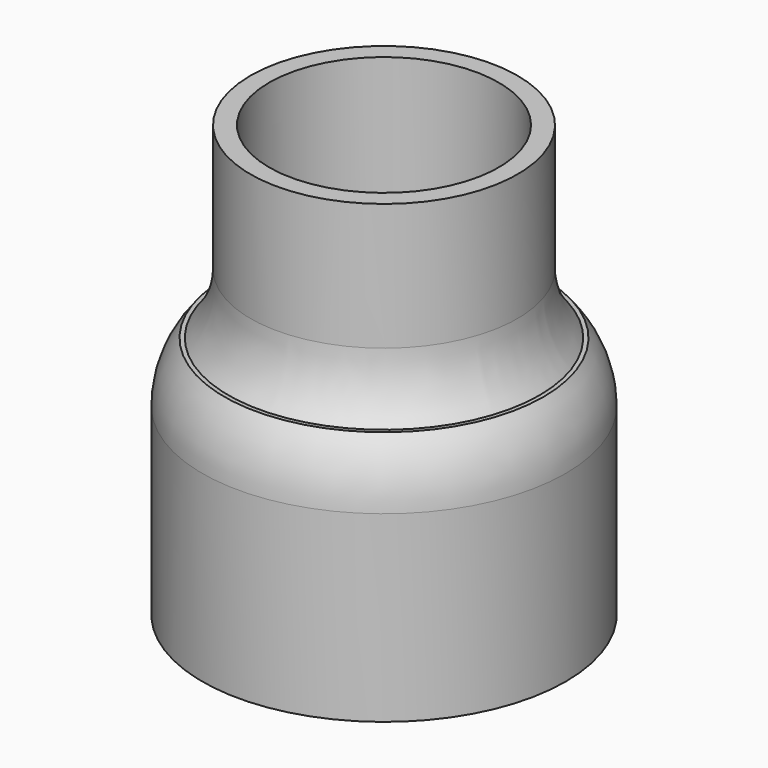
from build123d import *

# Parameters (mm, degrees)
F0_W    = 7.13
F0_H    = 10
F0_H_2  = 3
F2_T    = -1
F3_SIZE = 1.175
F4_SIZE = 1.175
F5_R    = 2


# Not quite as in the source:
# - a fillet or chamfer that OpenCascade refuses, or shapes differently, is made with other operations: its cross-section is extruded or revolved along the edge and cut away or added


with BuildPart() as f1:
    # F0 (on Front) → F1 (revolve)
    with BuildSketch(Plane.XZ):
        with Locations((-3.565, 8)):
            Rectangle(F0_W, F0_H)
        with Locations((-3.565, 1.5)):
            Rectangle(F0_W, F0_H_2)
        Polygon((0, -10), (0, 0), (-7.13, 0), (-7.13, 3), (-9.7, 3), (-9.7, -10), align=None)
    revolve(axis=Axis((0, 0, 6.5), (0, 0, 1)))

    # F2
    f2_openings = [f1.faces().sort_by_distance(p)[0] for p in [
        (0, 0, 13),
        (0, 0, -10),
    ]]
    offset(amount=F2_T, openings=f2_openings, kind=Kind.INTERSECTION)

    # F3
    f3_edges = [f1.edges().sort_by_distance(p)[0] for p in [
        (6.13, 0, 2),
        (-6.13, 0, 7.5),
        (8.7, 0, 2),
    ]]
    chamfer(f3_edges, length=F3_SIZE)

    # F4
    f4_edges = [f1.edges().sort_by_distance(p)[0] for p in [
        (9.7, 0, 3),
        (7.13, 0, 3),
    ]]
    chamfer(f4_edges, length=F4_SIZE)

    # F5
    f5_edges = [f1.edges().sort_by_distance(p)[0] for p in [
        (8.7, 0, 0.825),
    ]]
    fillet(f5_edges, radius=F5_R)

    # F6: fillet of radius 5 on 1 edges, made by hand

    # F6_s1 → F6_t2 (revolve)
    with BuildSketch(Plane.XZ):
        with BuildLine():
            ThreePointArc((-8.305, 3), (-7.432926443, 4.5062377439), (-7.13, 6.220151394))
            Line((-7.13, 6.220151394), (-7.13, 4.175))
            Line((-7.13, 4.175), (-8.305, 3))
        make_face()
    revolve(axis=Axis((0, 0, 4.175), (0, 0, 1)))

    # F7: fillet of radius 5 on 1 edges, made by hand

    # F7_s1 → F7_t2 (revolve, cut)
    with BuildSketch(Plane.XZ):
        with BuildLine():
            ThreePointArc((-9.7, -0.220151394), (-9.397073557, 1.4937622561), (-8.525, 3))
            Line((-8.525, 3), (-9.7, 1.825))
            Line((-9.7, 1.825), (-9.7, -0.220151394))
        make_face()
    revolve(axis=Axis((0, 0, 1.825), (0, 0, 1)), mode=Mode.SUBTRACT)


solid = f1.part
